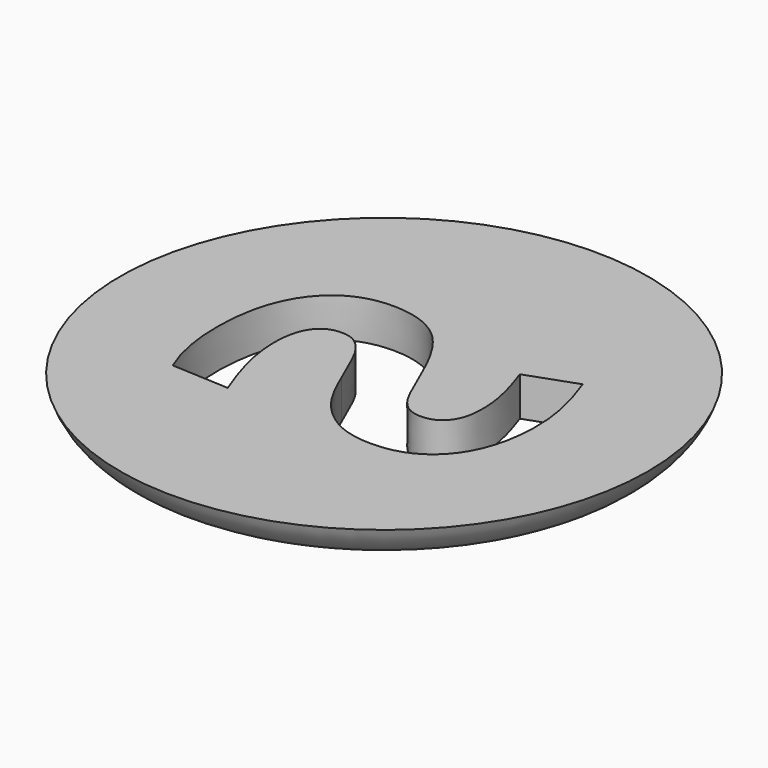
from build123d import *

# Parameters (mm, degrees)
F0_R         = 13.5
F1_DEPTH     = 2
F3_TEXT_SIZE = 20.8333333333
F4_DEPTH     = 2


# Not quite as in the source:
# - a fillet or chamfer that OpenCascade refuses, or shapes differently, is made with other operations: its cross-section is extruded or revolved along the edge and cut away or added
# - Text() gives the source's letters only with a copy of the font that has no kerning and outlines rounded to 1/6400 em; it was checked with that copy


with BuildPart() as f1:
    # F0 (on Top) → F1 (new body)
    with BuildSketch(Plane.XY):
        Circle(F0_R)
    extrude(amount=F1_DEPTH)

    # F2: fillet of radius 3 on 1 edges, made by hand

    # F2_s1 → F2_t2 (revolve, cut)
    with BuildSketch(Plane.XZ):
        with BuildLine():
            ThreePointArc((13.5, 2), (12.4036236828, 0.5505102572), (10.6715728753, 0))
            Line((10.6715728753, 0), (13.5, 0))
            Line((13.5, 0), (13.5, 2))
        make_face()
    revolve(axis=Axis((0, 0, 0), (0, 0, 1)), mode=Mode.SUBTRACT)

    # F3 (on face) → F4 (cut)
    with BuildSketch(Plane(origin=(0, 0, 0), x_dir=(1, 0, 0), z_dir=(0, 0, -1))):
        with Locations(Location((-7.7850712429, 5.6262230179), (0, 0, -87.1910506216))):
            Text('S', F3_TEXT_SIZE, font='Open Sans', font_style=FontStyle.BOLD, text_align=(TextAlign.LEFT, TextAlign.BOTTOM))
    extrude(amount=-F4_DEPTH, mode=Mode.SUBTRACT)


solid = f1.part
